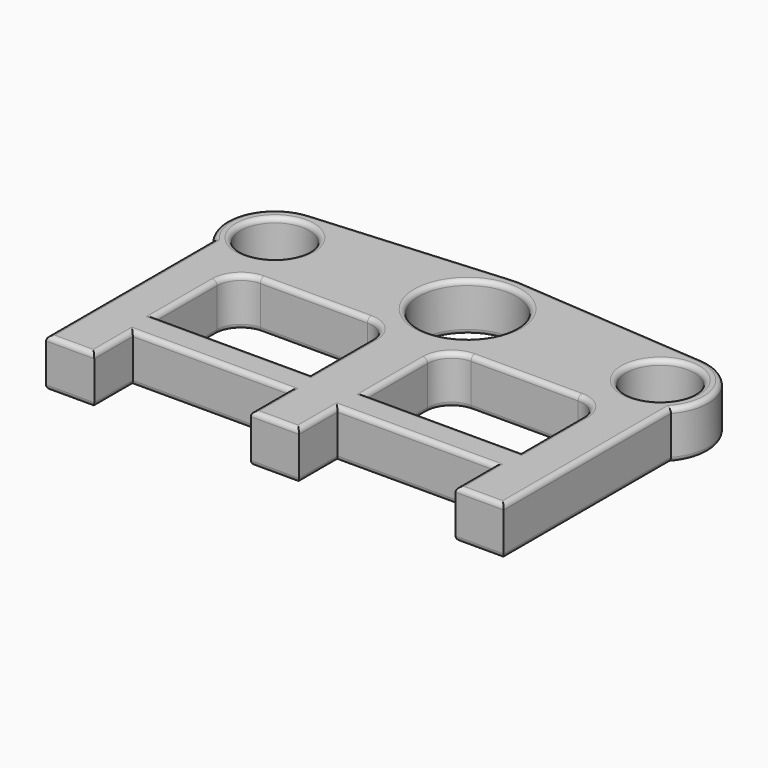
from build123d import *

# Parameters (mm, degrees)
F0_R     = 7.1
F0_R_2   = 10.1
F1_DEPTH = 10
F2_R     = 1


# Not quite as in the source:
# - a feature names something its author has since deleted; it is built from what else it names


with BuildPart() as f1:
    # F0 (on Top) → F1 (new body)
    with BuildSketch(Plane.XY):
        with BuildLine():
            Line((-37.5, -50), (-37.5, -40))
            Line((-37.5, -40), (-5, -40))
            Line((-5, -40), (-5, -50))
            Line((-5, -50), (0, -50))
            Line((0, -50), (5, -50))
            Line((5, -50), (5, -40))
            Line((5, -40), (37.5, -40))
            Line((37.5, -40), (37.5, -50))
            Line((37.5, -50), (47.5, -50))
            Line((47.5, -50), (47.5, -40))
            Line((47.5, -40), (47.5, -6.6143782777))
            ThreePointArc((47.5, -6.6143782777), (49.2623563699, 3.7694501558), (40.75, 9.9718353376))
            Line((40.75, 9.9718353376), (0.975, 12.9633859389))
            ThreePointArc((0.975, 12.9633859389), (0, 13), (-0.975, 12.9633859389))
            Line((-0.975, 12.9633859389), (-40.75, 9.9718353376))
            ThreePointArc((-40.75, 9.9718353376), (-49.2623563699, 3.7694501558), (-47.5, -6.6143782777))
            Line((-47.5, -6.6143782777), (-47.5, -40))
            Line((-47.5, -40), (-47.5, -50))
            Line((-47.5, -50), (-37.5, -50))
        make_face()
        with BuildLine():
            Line((-5.7514859363, -17.5539107248), (-5.7514859363, -33.6591888964))
            Line((-5.7514859363, -33.6591888964), (-37.9789326537, -33.6591888964))
            Line((-37.9789326537, -33.6591888964), (-37.9789326537, -17.5539107248))
            ThreePointArc((-37.9789326537, -17.5539107248), (-36.5144665596, -14.0183768189), (-32.9789326537, -12.5539107248))
            Line((-32.9789326537, -12.5539107248), (-10.7514859363, -12.5539107248))
            ThreePointArc((-10.7514859363, -12.5539107248), (-7.2159520304, -14.0183768189), (-5.7514859363, -17.5539107248))
        make_face(mode=Mode.SUBTRACT)
        with BuildLine():
            Line((37.9789326537, -33.6591888964), (5.7514859363, -33.6591888964))
            Line((5.7514859363, -33.6591888964), (5.7514859363, -17.5539107248))
            ThreePointArc((5.7514859363, -17.5539107248), (7.2159520304, -14.0183768189), (10.7514859363, -12.5539107248))
            Line((10.7514859363, -12.5539107248), (32.9789326537, -12.5539107248))
            ThreePointArc((32.9789326537, -12.5539107248), (36.5144665596, -14.0183768189), (37.9789326537, -17.5539107248))
            Line((37.9789326537, -17.5539107248), (37.9789326537, -33.6591888964))
        make_face(mode=Mode.SUBTRACT)
        with Locations((-40, 0)):
            Circle(F0_R, mode=Mode.SUBTRACT)
        Circle(F0_R_2, mode=Mode.SUBTRACT)
        with Locations((40, 0)):
            Circle(F0_R, mode=Mode.SUBTRACT)
    extrude(amount=F1_DEPTH)

    # F2
    f2_edges = [f1.edges().sort_by_distance(p)[0] for p in [
        (-49.262356, 3.76945, 10),
        (-47.5, -28.307189, 10),
        (-42.5, -50, 10),
        (-37.5, -45, 10),
        (-21.25, -40, 10),
        (-5, -45, 10),
        (0, -50, 10),
        (5, -45, 10),
        (21.25, -40, 10),
        (37.5, -45, 10),
        (42.5, -50, 10),
        (47.5, -28.307189, 10),
        (49.262356, 3.76945, 10),
        (20.8625, 11.467611, 10),
        (0, 13, 10),
        (-20.8625, 11.467611, 10),
        (-5.751486, -25.60655, 10),
        (-21.865209, -33.659189, 10),
        (-37.978933, -25.60655, 10),
        (-36.514467, -14.018377, 10),
        (-21.865209, -12.553911, 10),
        (-7.215952, -14.018377, 10),
        (37.978933, -25.60655, 10),
        (21.865209, -33.659189, 10),
        (5.751486, -25.60655, 10),
        (7.215952, -14.018377, 10),
        (21.865209, -12.553911, 10),
        (36.514467, -14.018377, 10),
        (-47.1, 0, 10),
        (-10.1, 0, 10),
        (32.9, 0, 10),
        (-49.262356, 3.76945, 0),
        (-47.5, -28.307189, 0),
        (-42.5, -50, 0),
        (-37.5, -45, 0),
        (-21.25, -40, 0),
        (-5, -45, 0),
        (0, -50, 0),
        (5, -45, 0),
        (21.25, -40, 0),
        (37.5, -45, 0),
        (42.5, -50, 0),
        (47.5, -28.307189, 0),
        (49.262356, 3.76945, 0),
        (20.8625, 11.467611, 0),
        (0, 13, 0),
        (-20.8625, 11.467611, 0),
        (-5.751486, -25.60655, 0),
        (-21.865209, -33.659189, 0),
        (-37.978933, -25.60655, 0),
        (-36.514467, -14.018377, 0),
        (-21.865209, -12.553911, 0),
        (-7.215952, -14.018377, 0),
        (37.978933, -25.60655, 0),
        (21.865209, -33.659189, 0),
        (5.751486, -25.60655, 0),
        (7.215952, -14.018377, 0),
        (21.865209, -12.553911, 0),
        (36.514467, -14.018377, 0),
        (-47.1, 0, 0),
        (-10.1, 0, 0),
        (32.9, 0, 0),
    ]]
    fillet(f2_edges, radius=F2_R)


solid = f1.part
